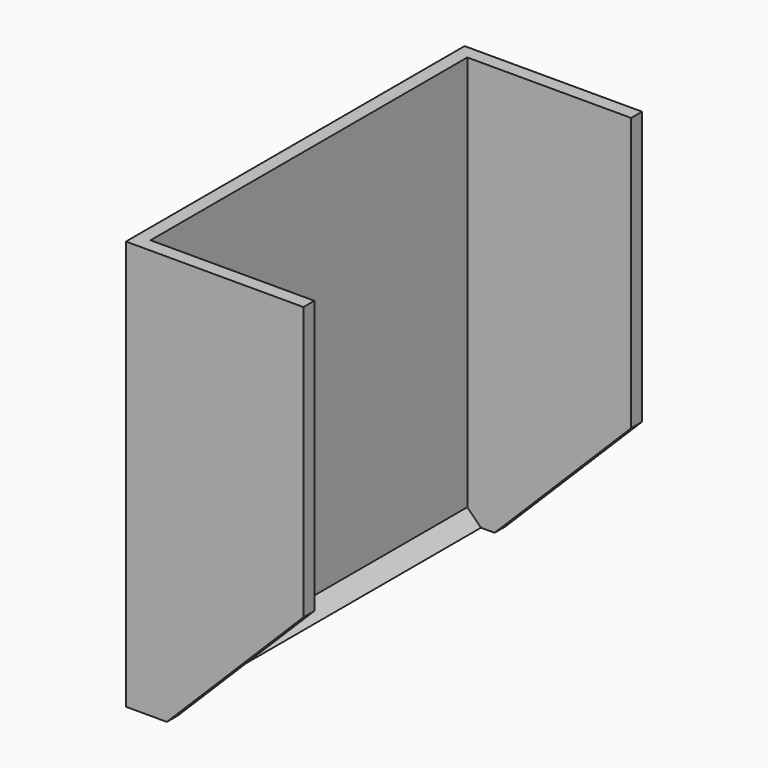
from build123d import *

# Parameters (mm, degrees)
F0_W        = 78.74
F0_H        = 76.2
F1_DEPTH    = 33.02
F2_T        = -2.54
F3_T4_DEPTH = 73.66
F4_SIZE     = 25.4


# Not quite as in the source:
# - a fillet or chamfer that OpenCascade refuses, or shapes differently, is made with other operations: its cross-section is extruded or revolved along the edge and cut away or added


with BuildPart() as f1:
    # F0 (on Right) → F1 (new body)
    with BuildSketch(Plane.YZ):
        with Locations((-1.4558544075, -12.2276971856)):
            Rectangle(F0_W, F0_H)
    extrude(amount=F1_DEPTH)

    # F2
    f2_openings = [f1.faces().sort_by_distance(p)[0] for p in [
        (33.02, -1.455854, -12.227697),
        (16.51, -1.455854, 25.872303),
    ]]
    offset(amount=F2_T, openings=f2_openings)

    # F3: chamfer of 30.48 on 1 edges, made by hand


with BuildPart() as f3_tool2:
    # F3_s3 → F3_t4 (new body)
    with BuildSketch(Plane.XZ.offset(38.2858544075)):
        with BuildLine():
            Line((33.8821045876, -79.1298017732), (1.6778954124, -46.925592598))
            Line((1.6778954124, -46.925592598), (1.6778954124, -46.315992598))
            ThreePointArc((1.6778954124, -46.315992598), (17.3489477062, -47.1780971856), (33.02, -47.1780971856))
            Line((33.02, -47.1780971856), (33.6296, -47.7876971856))
            ThreePointArc((33.6296, -47.7876971856), (33.6296, -63.4587494794), (34.4917045876, -79.1298017732))
            Line((34.4917045876, -79.1298017732), (33.8821045876, -79.1298017732))
        make_face()
    extrude(amount=-F3_T4_DEPTH)

    split(bisect_by=Plane.YZ.offset(2.54), keep=Keep.TOP)


with BuildPart() as f1_1:
    add(f1.part)

    # F3_t1: cut F3_tool2
    add(f3_tool2.part, mode=Mode.SUBTRACT)

    # F4
    f4_edges = [f1_1.edges().sort_by_distance(p)[0] for p in [
        (33.02, -39.555854, -50.327697),
        (33.02, 36.644146, -50.327697),
    ]]
    chamfer(f4_edges, length=F4_SIZE)


solid = f1_1.part
